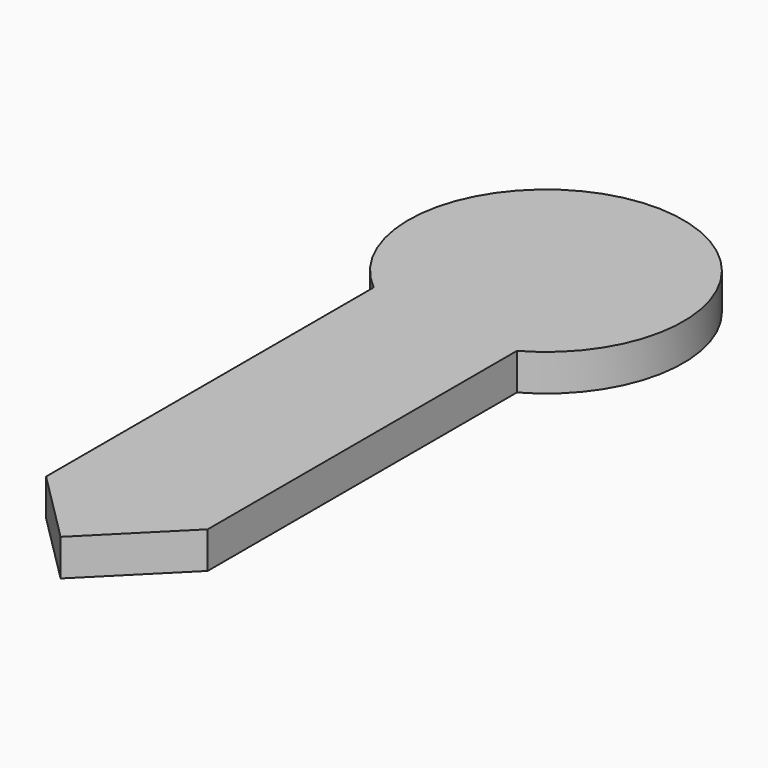
from build123d import *

# Parameters (mm, degrees)
F0_R        = 3.81
F1_DEPTH    = 1.016
F2_W        = 4.2779184878
F2_H        = 13.4340701625
F3_DEPTH    = 1.016
F4_SIZE     = 2.286
F5_T1_DEPTH = 11.4673196631


# Not quite as in the source:
# - a fillet or chamfer that OpenCascade refuses, or shapes differently, is made with other operations: its cross-section is extruded or revolved along the edge and cut away or added


with BuildPart() as f1:
    # F0 (on Top) → F1 (new body)
    with BuildSketch(Plane.XY):
        with Locations((-29.276387766, 26.0032489896)):
            Circle(F0_R)
    extrude(amount=F1_DEPTH)

    # F2 (on Top) → F3 (join)
    with BuildSketch(Plane.XY):
        with Locations((-29.5591074973, 16.392851714)):
            Rectangle(F2_W, F2_H)
    extrude(amount=F3_DEPTH)

    # F4
    f4_edges = [f1.edges().sort_by_distance(p)[0] for p in [
        (-27.420148, 9.675817, 0.508),
    ]]
    chamfer(f4_edges, length=F4_SIZE)

    # F5: chamfer of 2.032 on 1 edges, made by hand

    # F5_s2 → F5_t1 (cut)
    with BuildSketch(Plane.XY.offset(-5.2256598315)):
        Polygon((-29.6660667412, 9.6758166328), (-31.6980667412, 11.7078166328), (-31.6980667412, 9.6758166328), align=None)
    extrude(amount=F5_T1_DEPTH, mode=Mode.SUBTRACT)


solid = f1.part
